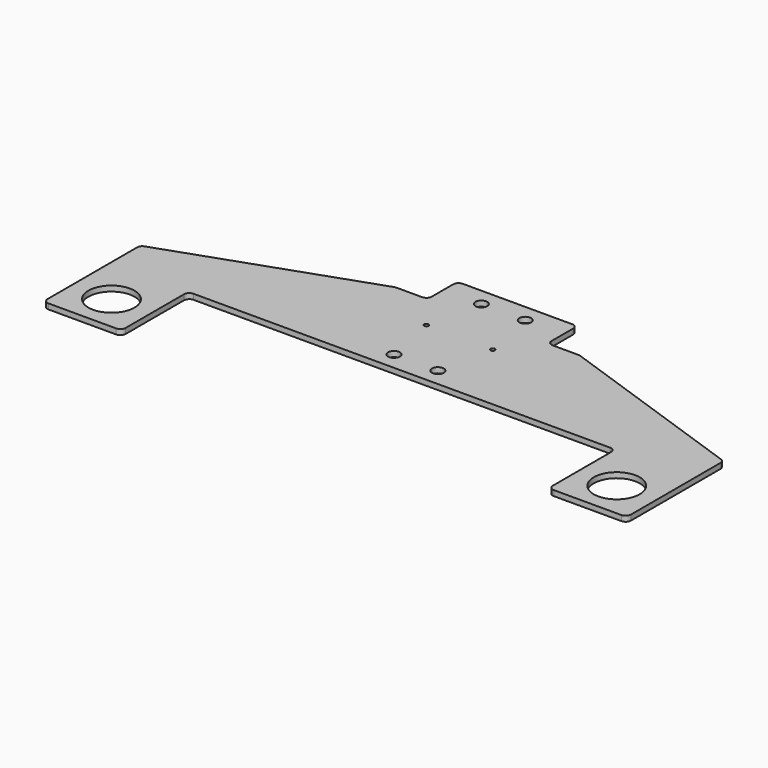
from build123d import *

# Parameters (mm, degrees)
F0_W     = 73
F0_H     = 78
F0_W_2   = 112
F0_H_2   = 35
F1_DEPTH = 5
F2_R     = 5
F3_R     = 5
F6_D     = 4.1
F8_D     = 43
F9_D     = 11


# Not quite as in the source:
# - a feature names something its author has since deleted; it is built from what else it names


with BuildPart() as f1:
    # F0 (on Top) → F1 (new body)
    with BuildSketch(Plane.XY):
        Polygon((-56, 50), (-86, 50), (-272.5, -15), (-272.5, -50), (-199.5, -50), (199.5, -50), (272.5, -50), (272.5, -15), (86, 50), (56, 50), align=None)
        with Locations((-236, -89)):
            Rectangle(F0_W, F0_H)
        with Locations((236, -89)):
            Rectangle(F0_W, F0_H)
        with Locations((0, 67.5)):
            Rectangle(F0_W_2, F0_H_2)
    extrude(amount=F1_DEPTH)

    # F2
    f2_edges = [f1.edges().sort_by_distance(p)[0] for p in [
        (-272.5, -128, 2.5),
        (-199.5, -128, 2.5),
        (199.5, -128, 2.5),
        (272.5, -128, 2.5),
        (272.5, -15, 2.5),
        (-272.5, -15, 2.5),
        (-199.5, -50, 2.5),
        (199.5, -50, 2.5),
        (-56, 50, 2.5),
        (-56, 85, 2.5),
        (56, 85, 2.5),
        (56, 50, 2.5),
    ]]
    fillet(f2_edges, radius=F2_R)

    # F3
    f3_edges = [f1.edges().sort_by_distance(p)[0] for p in [
        (86, 50, 2.5),
        (-86, 50, 2.5),
    ]]
    fillet(f3_edges, radius=F3_R)

    # F6 (through all)
    with Locations(Plane(origin=(0, 0, 0), x_dir=(1, 0, 0), z_dir=(0, 0, -1))):
        with Locations((-31, -17.5), (31, -17.5)):
            Hole(F6_D / 2)

    # F8 (through all)
    with Locations(Plane(origin=(0, 0, 0), x_dir=(1, 0, 0), z_dir=(0, 0, -1))):
        with Locations((-236, 94), (236, 94)):
            Hole(F8_D / 2)

    # F9 (through all)
    with Locations(Plane(origin=(0, 0, 0), x_dir=(1, 0, 0), z_dir=(0, 0, -1))):
        with Locations((-20.5, -68.5), (20.5, -68.5), (-20.5, 33.5), (20.5, 33.5)):
            Hole(F9_D / 2)


solid = f1.part
